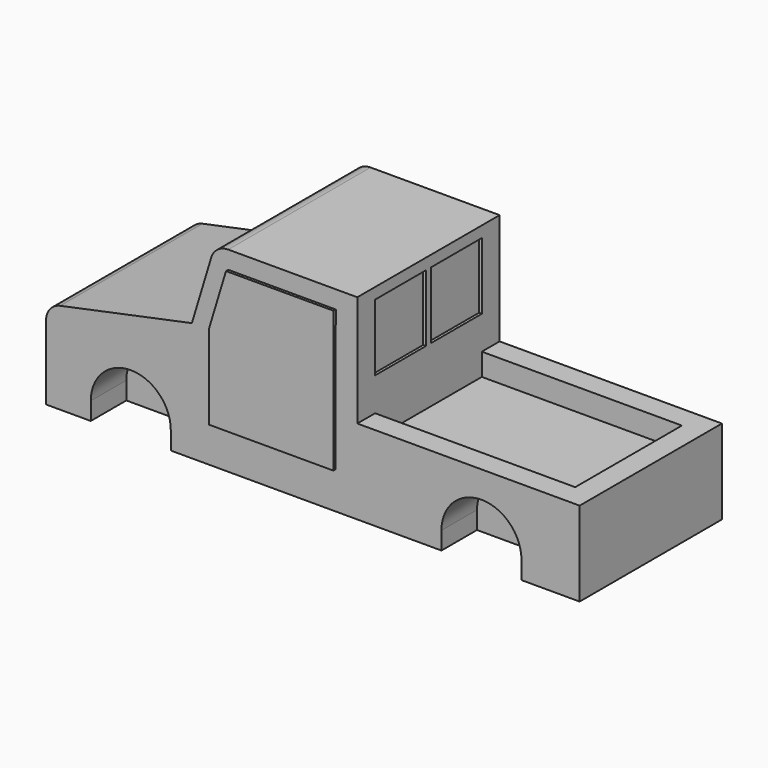
from build123d import *

# Parameters (mm, degrees)
F1_DEPTH    = 50.8
F2_W        = 57.15
F2_H        = 38.1
F3_DEPTH    = 6.35
F4_W        = 23.114
F4_H        = 6.604
F4_W_2      = 0.9801145643
F4_H_2      = 5.08
F5_DEPTH    = 2.54
F4_R        = 2.667
F6_DEPTH    = 1.27
F8_DEPTH    = 0.8001
F9_T1_DEPTH = 71.4372925246
F9_T3_DEPTH = 69.6542925277
F11_DEPTH   = 0.8001
F13_DEPTH   = 0.8001
F15_DEPTH   = 0.254
F16_W       = 18.161
F16_H       = 19.05
F17_DEPTH   = 0.8001
F18_DEPTH   = 50.8
F19_W       = 127
F19_H       = 25.4
F20_DEPTH   = 12.7
F21_DEPTH   = 5.08
F22_R       = 1.397
F23_R       = 1.397
F24_DEPTH   = 25.4


# Not quite as in the source:
# - a fillet or chamfer that OpenCascade refuses, or shapes differently, is made with other operations: its cross-section is extruded or revolved along the edge and cut away or added


with BuildPart() as f1:
    # F0 (on Front) → F1 (new body)
    with BuildSketch(Plane.XZ):
        with BuildLine():
            Line((-68.745650351, 20.2095657587), (-68.745650351, 0))
            Line((-68.745650351, 0), (-55.97953596, 0))
            ThreePointArc((-55.97953596, 0), (-44.54953596, 11.43), (-33.11953596, 0))
            Line((-33.11953596, 0), (44.1833575737, 0))
            ThreePointArc((44.1833575737, 0), (55.6133575737, 11.43), (67.0433575737, 0))
            Line((67.0433575737, 0), (83.654349649, 0))
            Line((83.654349649, 0), (83.654349649, 19.05))
            Line((83.654349649, 19.05), (20.154349649, 19.05))
            Line((20.154349649, 19.05), (20.154349649, 50.8))
            Line((20.154349649, 50.8), (-20.485650351, 50.8))
            Line((-20.485650351, 50.8), (-27.103371678, 28.9188353957))
            Line((-27.103371678, 28.9188353957), (-68.745650351, 20.2095657587))
        make_face()
        with BuildLine():
            ThreePointArc((-33.11953596, 0), (-44.54953596, 11.43), (-55.97953596, 0))
            Line((-55.97953596, 0), (-33.11953596, 0))
        make_face()
        with BuildLine():
            ThreePointArc((67.0433575737, 0), (55.6133575737, 11.43), (44.1833575737, 0))
            Line((44.1833575737, 0), (67.0433575737, 0))
        make_face()
    extrude(amount=F1_DEPTH)

    # F2 (on face) → F3 (cut)
    with BuildSketch(Plane.XY.offset(19.05)):
        with Locations((48.729349649, -25.4)):
            Rectangle(F2_W, F2_H)
    extrude(amount=-F3_DEPTH, mode=Mode.SUBTRACT)

    # F4 (on face) → F5 (join)
    with BuildSketch(Plane(origin=(-68.745650351, 0, 0), x_dir=(0, -1, 0), z_dir=(-1, 0, 0))):
        with Locations((25.4, 9.8053713022)):
            Rectangle(F4_W, F4_H)
        Polygon((36.195, 12.3453713022), (36.195, 7.2653713022), (32.6746520766, 7.2653713022), (31.6945375124, 7.2653713022), (29.2964520766, 7.2653713022), (28.3163375124, 7.2653713022), (25.9182520766, 7.2653713022), (24.9381375124, 7.2653713022), (22.5400520766, 7.2653713022), (21.5599375124, 7.2653713022), (19.1618520766, 7.2653713022), (18.1817375124, 7.2653713022), (14.605, 7.2653713022), (14.605, 12.3453713022), (18.1817375124, 12.3453713022), (19.1618520766, 12.3453713022), (21.5599375124, 12.3453713022), (22.5400520766, 12.3453713022), (24.9381375124, 12.3453713022), (25.9182520766, 12.3453713022), (28.3163375124, 12.3453713022), (29.2964520766, 12.3453713022), (31.6945375124, 12.3453713022), (32.6746520766, 12.3453713022), align=None, mode=Mode.SUBTRACT)
        with Locations((18.6717947945, 9.8053713022)):
            Rectangle(F4_W_2, F4_H_2)
        with Locations((22.0499947945, 9.8053713022)):
            Rectangle(F4_W_2, F4_H_2)
        with Locations((25.4281947945, 9.8053713022)):
            Rectangle(F4_W_2, F4_H_2)
        with Locations((28.8063947945, 9.8053713022)):
            Rectangle(F4_W_2, F4_H_2)
        with Locations((32.1845947945, 9.8053713022)):
            Rectangle(F4_W_2, F4_H_2)
    extrude(amount=F5_DEPTH)

    # F4 (on face) → F6 (join)
    with BuildSketch(Plane(origin=(-68.745650351, 0, 0), x_dir=(0, -1, 0), z_dir=(-1, 0, 0))):
        with Locations((6.35, 9.8351975903)):
            Circle(F4_R)
        with Locations((44.45, 9.8351975903)):
            Circle(F4_R)
    extrude(amount=F6_DEPTH)

    # F7 (on face) → F8 (cut)
    with BuildSketch(Plane(origin=(-32.8452255156, 0, 9.9336828416), x_dir=(0, -1, 0), z_dir=(-0.9571813038, 0, 0.2894891219))):
        Polygon((33.562220633, 22.6956736296), (47.9775152107, 22.6956736296), (47.9775152107, 40.2216736296), (2.2575152107, 40.2216736296), (2.2575152107, 22.6956736296), (16.4677330811, 22.6956736296), (15.0759897713, 29.1358400136), (13.6842464615, 33.1220440567), (16.4677330811, 29.1358400136), (17.814220633, 22.6956736296), (32.2157330811, 22.6956736296), (30.8239897713, 29.1358400136), (29.4322464615, 33.1220440567), (32.2157330811, 29.1358400136), align=None)
    extrude(amount=-F8_DEPTH, mode=Mode.SUBTRACT)

    # F9: fillet of radius 5.08 on 2 edges, made by hand

    # F9_s2 → F9_t1 (cut)
    with BuildSketch(Plane.XZ.offset(-10.3186462623)):
        with BuildLine():
            ThreePointArc((-64.7056051643, 21.0545205498), (-67.6083252331, 19.2854983904), (-68.745650351, 16.0821072538))
            Line((-68.745650351, 16.0821072538), (-68.745650351, 20.2095657587))
            Line((-68.745650351, 20.2095657587), (-64.7056051643, 21.0545205498))
        make_face()
    extrude(amount=F9_T1_DEPTH, mode=Mode.SUBTRACT)

    # F9_s4 → F9_t3 (cut)
    with BuildSketch(Plane.XZ.offset(-9.4271462638)):
        with BuildLine():
            ThreePointArc((-21.5772728687, 47.1906047393), (-19.74263992, 49.7990361653), (-16.7147918455, 50.8))
            Line((-16.7147918455, 50.8), (-20.485650351, 50.8))
            Line((-20.485650351, 50.8), (-21.5772728687, 47.1906047393))
        make_face()
    extrude(amount=F9_T3_DEPTH, mode=Mode.SUBTRACT)

    # F10 (on face) → F11 (join)
    with BuildSketch(Plane.XZ.offset(50.8)):
        Polygon((13.9938081476, 45.7206499122), (-16.7147918455, 45.72), (-21.5772728687, 29.6424496777), (-21.5772728687, 5.5124496777), (13.9827271313, 5.5124514391), align=None)
    extrude(amount=F11_DEPTH)

    # F12 (on face) → F13 (join)
    with BuildSketch(Plane(origin=(0, 0, 0), x_dir=(-1, 0, 0), z_dir=(0, 1, 0))):
        Polygon((21.566192252, 29.6467966337), (16.7147918455, 45.72), (-13.993807748, 45.7249966337), (-13.993807748, 5.5167966337), (21.566192252, 5.5167966337), align=None)
    extrude(amount=F13_DEPTH)

    # F14 (on face) → F15 (join)
    with BuildSketch(Plane(origin=(0, 0.8001, 0), x_dir=(-1, 0, 0), z_dir=(0, 1, 0))):
        Polygon((-11.5635488182, 29.6467966337), (18.8161898404, 29.6467966337), (14.9059221148, 43.1567057967), (-11.5635488182, 43.1567057967), align=None)
    extrude(amount=-F15_DEPTH)

    # F16 (on face) → F17 (cut)
    with BuildSketch(Plane.YZ.offset(20.154349649)):
        with Locations((-35.3695, 38.1)):
            Rectangle(F16_W, F16_H)
        with Locations((-15.4305, 38.1)):
            Rectangle(F16_W, F16_H)
    extrude(amount=-F17_DEPTH, mode=Mode.SUBTRACT)

    # F0 (on Front) → F18 (cut)
    with BuildSketch(Plane.XZ):
        with BuildLine():
            ThreePointArc((67.0433575737, 0), (55.6133575737, 11.43), (44.1833575737, 0))
            Line((44.1833575737, 0), (67.0433575737, 0))
        make_face()
        with BuildLine():
            ThreePointArc((-33.11953596, 0), (-44.54953596, 11.43), (-55.97953596, 0))
            Line((-55.97953596, 0), (-33.11953596, 0))
        make_face()
    extrude(amount=F18_DEPTH, mode=Mode.SUBTRACT)

    # F19 (on face) → F20 (join)
    with BuildSketch(Plane(origin=(0, 0, 0), x_dir=(1, 0, 0), z_dir=(0, 0, -1))):
        with Locations((6.3173042834, 25.4)):
            Rectangle(F19_W, F19_H)
    extrude(amount=-F20_DEPTH)

    # F21 (add): a face of the model
    f21_faces = [f1.faces().sort_by_distance(p)[0] for p in [
        (7.7936035623, -25.4, 0),
    ]]
    extrude(f21_faces, amount=F21_DEPTH)

    # F22 (on face) + F23 (on face) → F24 (cut)
    with BuildSketch(Plane(origin=(0, -12.7, 0), x_dir=(-1, 0, 0), z_dir=(0, 1, 0))):
        with Locations((-55.6133575737, 0)):
            Circle(F22_R)
    with BuildSketch(Plane(origin=(0, -12.7, 0), x_dir=(-1, 0, 0), z_dir=(0, 1, 0))):
        with Locations((44.54953596, 0)):
            Circle(F23_R)
    extrude(amount=-F24_DEPTH, mode=Mode.SUBTRACT)


solid = f1.part
